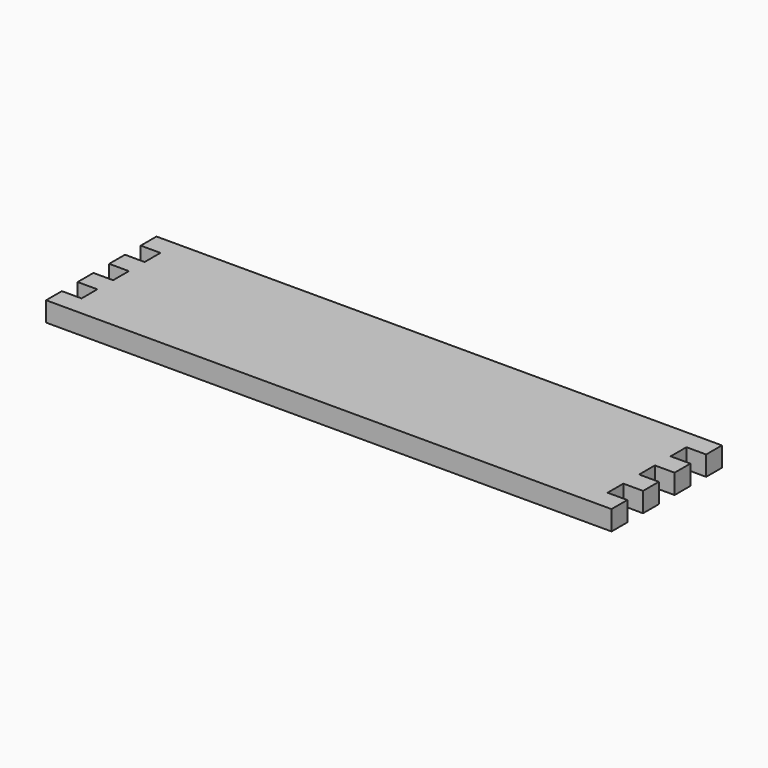
from build123d import *

# Parameters (mm, degrees)
F0_W     = 10
F0_H     = 10
F1_DEPTH = 10


# Not quite as in the source:
# - a feature names something its author has since deleted; it is built from what else it names


with BuildPart() as f1:
    # F0 (on Top) → F1 (new body)
    with BuildSketch(Plane.XY):
        Polygon((131.1653250098, 36.9413525529), (-135.6346749902, 36.9413525529), (-135.6346749902, 26.9413525529), (-135.6346749902, 16.9413525529), (-135.6346749902, 6.9413525529), (-135.6346749902, -3.0586474471), (-135.6346749902, -13.0586474471), (-135.6346749902, -23.0586474471), (-135.6346749902, -33.0586474471), (131.1653250098, -33.0586474471), (131.1653250098, -23.0586474471), (131.1653250098, -13.0586474471), (131.1653250098, -3.0586474471), (131.1653250098, 6.9413525529), (131.1653250098, 16.9413525529), (131.1653250098, 26.9413525529), align=None)
        with Locations((-140.6346749902, 31.9413525529)):
            Rectangle(F0_W, F0_H)
        with Locations((-140.6346749902, 11.9413525529)):
            Rectangle(F0_W, F0_H)
        with Locations((-140.6346749902, -8.0586474471)):
            Rectangle(F0_W, F0_H)
        with Locations((-140.6346749902, -28.0586474471)):
            Rectangle(F0_W, F0_H)
        with Locations((136.1653250098, 31.9413525529)):
            Rectangle(F0_W, F0_H)
        with Locations((136.1653250098, 11.9413525529)):
            Rectangle(F0_W, F0_H)
        with Locations((136.1653250098, -8.0586474471)):
            Rectangle(F0_W, F0_H)
        with Locations((136.1653250098, -28.0586474471)):
            Rectangle(F0_W, F0_H)
    extrude(amount=F1_DEPTH)


solid = f1.part
